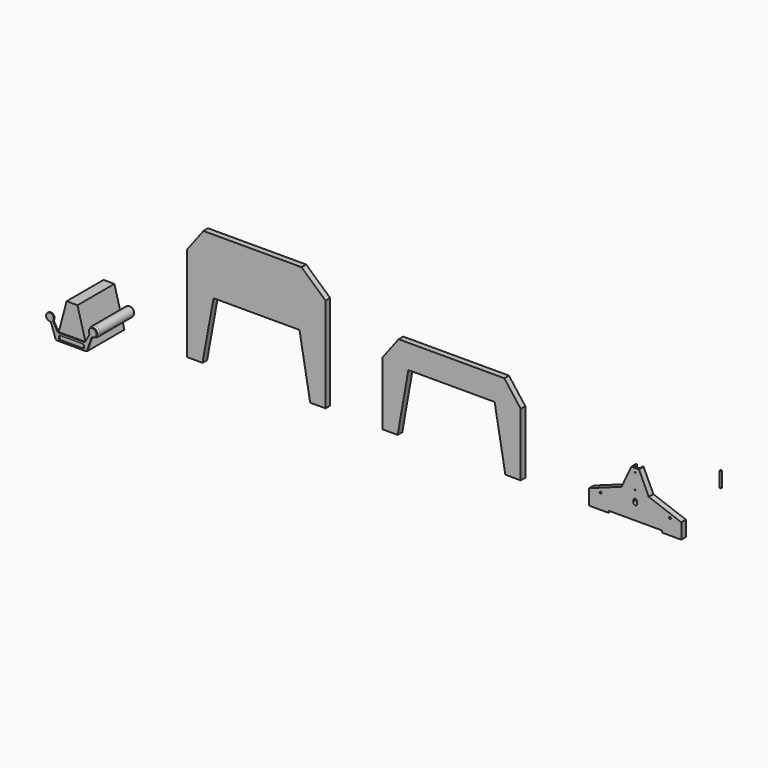
from build123d import *

# Parameters (mm, degrees)
F1_DEPTH  = 19.05
F2_R      = 3.175
F3_DEPTH  = 19.05
F4_W      = 19.05
F4_H      = 88.9
F5_DEPTH  = 12.7
F6_R      = 1.5875
F7_DEPTH  = 6.35
F8_R      = 3.175
F9_DEPTH  = 50.8
F10_SIZE  = 0.79375
F12_DEPTH = 152.4
F13_W     = 82.55
F13_H     = 15.0095159877
F14_DEPTH = 3.175
F15_R     = 5.08
F16_R     = 15.875
F17_DEPTH = 152.4
F18_R     = 6.35


# Not quite as in the source:
# - a feature names something its author has since deleted; it is built from what else it names


with BuildPart() as f1:
    # F0 (on Front) → F1 (new body)
    with BuildSketch(Plane.XZ):
        Polygon((106.1141828492, 11.5090513026), (141.3994925511, -188.6038841095), (192.1994925511, -188.6038841095), (192.1994925511, 124.7630377858), (112.8244925511, 196.2005377858), (-211.0255074489, 196.2005377858), (-265.0005074489, 124.7630377858), (-265.0005074489, -188.3859314735), (-214.2005074489, -188.3859314735), (-177.7007011349, 11.5090513026), align=None)
    extrude(amount=F1_DEPTH)


with BuildPart() as f1b:
    # F0 (on Front) → F1, piece 2 (new body)
    with BuildSketch(Plane.XZ):
        Polygon((750.637189092, 11.7211622333), (785.922498794, -188.3917731787), (836.722498794, -188.3917731787), (836.722498794, 19.5707268213), (782.7483080176, 91.0088382275), (433.4982512736, 91.0127944155), (379.522498794, 19.5765685265), (379.522498794, -188.3859314735), (430.322498794, -188.3859314735), (465.6409224309, 11.7211622333), align=None)
    extrude(amount=F1_DEPTH)


with BuildPart() as f1c:
    # F0 (on Front) → F1, piece 3 (new body)
    with BuildSketch(Plane.XZ):
        Polygon((1062.3789626762, -137.6629166841), (1062.3789626762, -188.4629166841), (1125.8789626762, -188.4629166841), (1125.8789626762, -182.1129166841), (1303.4997188771, -182.1129166841), (1303.4997188771, -188.4629166841), (1366.9997188771, -188.4629166841), (1366.9997188771, -137.6629166841), (1259.5928523213, -98.570014302), (1227.3893407766, -29.5093609298), (1201.9893407766, -29.5093609298), (1169.785829232, -98.570014302), align=None)
    extrude(amount=F1_DEPTH)

    # F2 (on face) → F3 (cut, through all)
    with BuildSketch(Plane.XZ.offset(19.05)):
        with Locations((1100.8384227753, -137.6629166841)):
            Circle(F2_R)
        with Locations((1329.4384227753, -137.6629166841)):
            Circle(F2_R)
        with BuildLine():
            ThreePointArc((1209.190112656, -128.1379166841), (1213.0458730336, -137.446545681), (1221.03937397, -131.3129166841))
            ThreePointArc((1221.03937397, -131.3129166841), (1220.823002967, -129.6694157477), (1220.1886352841, -128.1379166841))
            ThreePointArc((1220.1886352841, -128.1379166841), (1214.68937397, -131.3129166841), (1209.190112656, -128.1379166841))
        make_face()
        with BuildLine():
            ThreePointArc((1209.190112656, -128.1379166841), (1214.68937397, -131.3129166841), (1220.1886352841, -128.1379166841))
            ThreePointArc((1220.1886352841, -128.1379166841), (1214.68937397, -124.9629166841), (1209.190112656, -128.1379166841))
        make_face()
        with BuildLine():
            ThreePointArc((1209.190112656, -128.1379166841), (1214.68937397, -124.9629166841), (1220.1886352841, -128.1379166841))
            ThreePointArc((1220.1886352841, -128.1379166841), (1220.823002967, -126.6064176205), (1221.03937397, -124.9629166841))
            ThreePointArc((1221.03937397, -124.9629166841), (1213.0458730336, -118.8292876871), (1209.190112656, -128.1379166841))
        make_face()
    extrude(amount=-F3_DEPTH, mode=Mode.SUBTRACT)

    # F4 (on face) → F5 (cut)
    with BuildSketch(Plane(origin=(0, 0, 0), x_dir=(-1, 0, 0), z_dir=(0, 1, 0))):
        with Locations((-1214.6893407766, -73.9593609298)):
            Rectangle(F4_W, F4_H)
    extrude(amount=-F5_DEPTH, mode=Mode.SUBTRACT)

    # F6 (on face) → F7 (cut, through all)
    with BuildSketch(Plane(origin=(0, -12.7, 0), x_dir=(-1, 0, 0), z_dir=(0, 1, 0))):
        with Locations((-1214.6893407766, -42.2093609298)):
            Circle(F6_R)
        with Locations((-1214.6893407766, -93.0093609298)):
            Circle(F6_R)
    extrude(amount=-F7_DEPTH, mode=Mode.SUBTRACT)


with BuildPart() as f9:
    # F8 (on Top) → F9 (new body)
    with BuildSketch(Plane.XY):
        with Locations((1491.4883375168, -11.9951693341)):
            Circle(F8_R)
    extrude(amount=F9_DEPTH)

    # F10
    f10_edges = [f9.edges().sort_by_distance(p)[0] for p in [
        (1488.313338, -11.995169, 50.8),
        (1488.313338, -11.995169, 0),
    ]]
    chamfer(f10_edges, length=F10_SIZE)


with BuildPart() as f12:
    # F11 (on Front) → F12 (new body)
    with BuildSketch(Plane.XZ):
        Polygon((-589.0208482742, -188.8071298599), (-487.4208482742, -188.8071298599), (-520.2908670023, -66.1345499212), (-556.1508295462, -66.1345499212), align=None)
    extrude(amount=F12_DEPTH)


with BuildPart() as f14:
    # F13 (on face) → F14 (new body)
    with BuildSketch(Plane.XZ.offset(152.4)):
        with BuildLine():
            Line((-606.1395994957, -140.3661550864), (-589.0208482742, -188.8071298599))
            Line((-589.0208482742, -188.8071298599), (-487.4208482742, -188.8071298599))
            Line((-487.4208482742, -188.8071298599), (-470.3020970528, -140.3661550864))
            ThreePointArc((-470.3020970528, -140.3661550864), (-460.941969274, -117.143187727), (-477.4715221366, -135.9498909781))
            Line((-477.4715221366, -135.9498909781), (-493.9948520198, -164.2726138722))
            Line((-493.9948520198, -164.2726138722), (-582.4468445286, -164.2726138722))
            Line((-582.4468445286, -164.2726138722), (-598.9701744119, -135.9498909781))
            ThreePointArc((-598.9701744119, -135.9498909781), (-615.4997272745, -117.143187727), (-606.1395994957, -140.3661550864))
        make_face()
        with Locations((-537.6746112347, -178.1273718661)):
            Rectangle(F13_W, F13_H, mode=Mode.SUBTRACT)
    extrude(amount=F14_DEPTH)

    # F15
    f15_edges = [f14.edges().sort_by_distance(p)[0] for p in [
        (-598.970174, -153.9875, -135.949891),
        (-606.139599, -153.9875, -140.366155),
        (-582.446845, -153.9875, -164.272614),
        (-589.020848, -153.9875, -188.80713),
        (-578.949611, -153.9875, -170.622614),
        (-578.949611, -153.9875, -185.63213),
        (-496.399611, -153.9875, -170.622614),
        (-496.399611, -153.9875, -185.63213),
        (-493.994852, -153.9875, -164.272614),
        (-487.420848, -153.9875, -188.80713),
        (-470.302097, -153.9875, -140.366155),
        (-477.471522, -153.9875, -135.949891),
    ]]
    fillet(f15_edges, radius=F15_R)


with BuildPart() as f17:
    # F16 (on face) → F17 (new body)
    with BuildSketch(Plane(origin=(0, -152.4, 0), x_dir=(-1, 0, 0), z_dir=(0, 1, 0))):
        with Locations((467.6027211189, -127.9563456774)):
            Circle(F16_R)
    extrude(amount=F17_DEPTH)

    # F18
    f18_edges = [f17.edges().sort_by_distance(p)[0] for p in [
        (-451.727721, -152.4, -127.956346),
        (-451.727721, 0, -127.956346),
    ]]
    fillet(f18_edges, radius=F18_R)


solid = Compound([f1.part, f1b.part, f1c.part, f9.part, f12.part, f14.part, f17.part])
